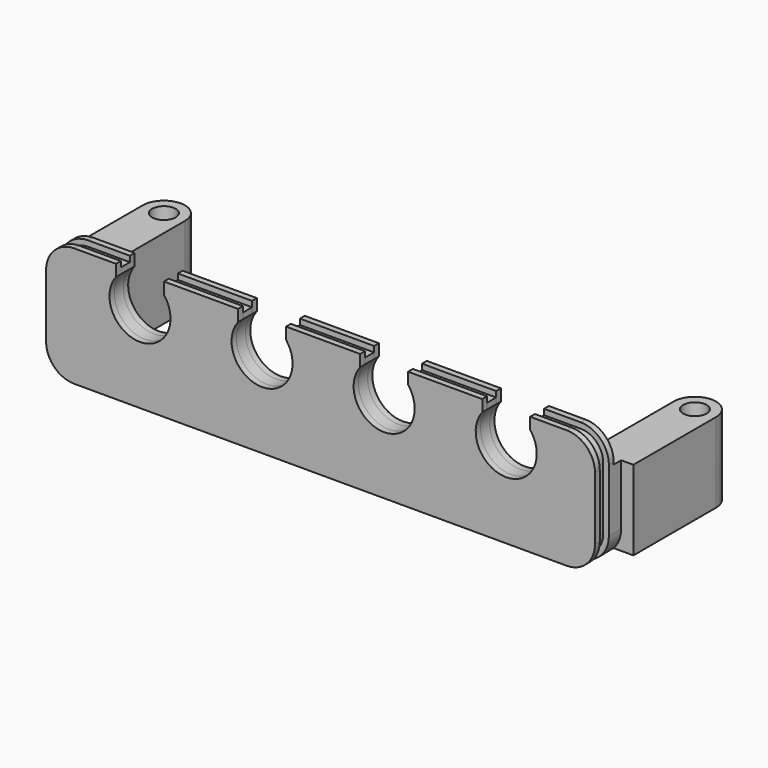
from build123d import *
from build123d import SkipClean  # not in build123d's __all__

# Parameters (mm, degrees)
F1_DEPTH = 0.64
F3_DEPTH = 1.21
F5_DEPTH = 0.64
F7_R     = 1.25
F8_DEPTH = 8.5
F9_DEPTH = 1


# Not quite as in the source:
# - after a boolean that leaves OpenCascade's solid faulty, fix() repairs it


with BuildPart() as f1:
    # F0 (on Front) → F1 (new body)
    with BuildSketch(Plane.XZ):
        with BuildLine():
            ThreePointArc((-29.225, -3.35), (-28.3463203436, -5.4713203436), (-26.225, -6.35))
            Line((-26.225, -6.35), (26.225, -6.35))
            ThreePointArc((26.225, -6.35), (28.3463203436, -5.4713203436), (29.225, -3.35))
            Line((29.225, -3.35), (29.225, 3.35))
            ThreePointArc((29.225, 3.35), (28.3463203436, 5.4713203436), (26.225, 6.35))
            Line((26.225, 6.35), (22.325, 6.35))
            Line((22.325, 6.35), (22.325, 5.114944168))
            ThreePointArc((22.325, 5.114944168), (19.775, -0.15), (17.225, 5.114944168))
            Line((17.225, 5.114944168), (17.225, 6.35))
            Line((17.225, 6.35), (9.325, 6.35))
            Line((9.325, 6.35), (9.325, 5.114944168))
            ThreePointArc((9.325, 5.114944168), (6.775, -0.15), (4.225, 5.114944168))
            Line((4.225, 5.114944168), (4.225, 6.35))
            Line((4.225, 6.35), (-3.675, 6.35))
            Line((-3.675, 6.35), (-3.675, 5.114944168))
            ThreePointArc((-3.675, 5.114944168), (-6.225, -0.15), (-8.775, 5.114944168))
            Line((-8.775, 5.114944168), (-8.775, 6.35))
            Line((-8.775, 6.35), (-16.675, 6.35))
            Line((-16.675, 6.35), (-16.675, 5.114944168))
            ThreePointArc((-16.675, 5.114944168), (-19.225, -0.15), (-21.775, 5.114944168))
            Line((-21.775, 5.114944168), (-21.775, 6.35))
            Line((-21.775, 6.35), (-26.225, 6.35))
            ThreePointArc((-26.225, 6.35), (-28.3463203436, 5.4713203436), (-29.225, 3.35))
            Line((-29.225, 3.35), (-29.225, -3.35))
        make_face()
    extrude(amount=-F1_DEPTH)

    # F2 (on face) → F3 (join)
    with BuildSketch(Plane(origin=(0, 0.64, 0), x_dir=(-1, 0, 0), z_dir=(0, 1, 0))):
        with BuildLine():
            Line((-22.325, 5.114944168), (-22.325, 5.75))
            Line((-22.325, 5.75), (-26.225, 5.75))
            ThreePointArc((-26.225, 5.75), (-27.9220562748, 5.0470562748), (-28.625, 3.35))
            Line((-28.625, 3.35), (-28.625, -3.35))
            ThreePointArc((-28.625, -3.35), (-27.9220562748, -5.0470562748), (-26.225, -5.75))
            Line((-26.225, -5.75), (26.225, -5.75))
            ThreePointArc((26.225, -5.75), (27.9220562748, -5.0470562748), (28.625, -3.35))
            Line((28.625, -3.35), (28.625, 3.35))
            ThreePointArc((28.625, 3.35), (27.9220562748, 5.0470562748), (26.225, 5.75))
            Line((26.225, 5.75), (21.775, 5.75))
            Line((21.775, 5.75), (21.775, 5.114944168))
            ThreePointArc((21.775, 5.114944168), (19.225, -0.15), (16.675, 5.114944168))
            Line((16.675, 5.114944168), (16.675, 5.75))
            Line((16.675, 5.75), (8.775, 5.75))
            Line((8.775, 5.75), (8.775, 5.114944168))
            ThreePointArc((8.775, 5.114944168), (6.225, -0.15), (3.675, 5.114944168))
            Line((3.675, 5.114944168), (3.675, 5.75))
            Line((3.675, 5.75), (-4.225, 5.75))
            Line((-4.225, 5.75), (-4.225, 5.114944168))
            ThreePointArc((-4.225, 5.114944168), (-6.775, -0.15), (-9.325, 5.114944168))
            Line((-9.325, 5.114944168), (-9.325, 5.75))
            Line((-9.325, 5.75), (-17.225, 5.75))
            Line((-17.225, 5.75), (-17.225, 5.114944168))
            ThreePointArc((-17.225, 5.114944168), (-19.775, -0.15), (-22.325, 5.114944168))
        make_face()
    with SkipClean():  # cleaning this boolean's faces spoils the solid; the shape is the same uncleaned
        extrude(amount=F3_DEPTH)

    # F4 (on face) → F5 (join)
    with BuildSketch(Plane(origin=(0, 1.85, 0), x_dir=(-1, 0, 0), z_dir=(0, 1, 0))):
        with BuildLine():
            ThreePointArc((-29.225, -3.35), (-28.3463203436, -5.4713203436), (-26.225, -6.35))
            Line((-26.225, -6.35), (26.225, -6.35))
            ThreePointArc((26.225, -6.35), (28.3463203436, -5.4713203436), (29.225, -3.35))
            Line((29.225, -3.35), (29.225, 3.35))
            ThreePointArc((29.225, 3.35), (28.3463203436, 5.4713203436), (26.225, 6.35))
            Line((26.225, 6.35), (21.775, 6.35))
            Line((21.775, 6.35), (21.775, 5.114944168))
            ThreePointArc((21.775, 5.114944168), (19.225, -0.15), (16.675, 5.114944168))
            Line((16.675, 5.114944168), (16.675, 6.35))
            Line((16.675, 6.35), (8.775, 6.35))
            Line((8.775, 6.35), (8.775, 5.114944168))
            ThreePointArc((8.775, 5.114944168), (6.225, -0.15), (3.675, 5.114944168))
            Line((3.675, 5.114944168), (3.675, 6.35))
            Line((3.675, 6.35), (-4.225, 6.35))
            Line((-4.225, 6.35), (-4.225, 5.114944168))
            ThreePointArc((-4.225, 5.114944168), (-6.775, -0.15), (-9.325, 5.114944168))
            Line((-9.325, 5.114944168), (-9.325, 6.35))
            Line((-9.325, 6.35), (-17.225, 6.35))
            Line((-17.225, 6.35), (-17.225, 5.114944168))
            ThreePointArc((-17.225, 5.114944168), (-19.775, -0.15), (-22.325, 5.114944168))
            Line((-22.325, 5.114944168), (-22.325, 6.35))
            Line((-22.325, 6.35), (-26.225, 6.35))
            ThreePointArc((-26.225, 6.35), (-28.3463203436, 5.4713203436), (-29.225, 3.35))
            Line((-29.225, 3.35), (-29.225, -3.35))
        make_face()
    extrude(amount=F5_DEPTH)

    add(f1.part.fix(), mode=Mode.REPLACE)

    # F7 (on offset) → F8 (join)
    with BuildSketch(Plane(origin=(0, 0, -5.4), x_dir=(1, 0, 0), z_dir=(0, 0, -1))):
        with BuildLine():
            Line((29.225, -3.49), (29.225, -2.49))
            Line((29.225, -2.49), (26.025, -2.49))
            Line((26.025, -2.49), (26.025, -3.49))
            Line((26.025, -3.49), (26.025, -14.49))
            ThreePointArc((26.025, -14.49), (28.275, -16.74), (30.525, -14.49))
            Line((30.525, -14.49), (30.525, -3.49))
            Line((30.525, -3.49), (29.225, -3.49))
        make_face()
        with Locations((28.275, -14.49)):
            Circle(F7_R, mode=Mode.SUBTRACT)
        with BuildLine():
            Line((-26.025, -14.49), (-26.025, -3.49))
            Line((-26.025, -3.49), (-26.025, -2.49))
            Line((-26.025, -2.49), (-29.225, -2.49))
            Line((-29.225, -2.49), (-29.225, -3.49))
            Line((-29.225, -3.49), (-30.525, -3.49))
            Line((-30.525, -3.49), (-30.525, -14.49))
            ThreePointArc((-30.525, -14.49), (-28.275, -16.74), (-26.025, -14.49))
        make_face()
        with Locations((-28.275, -14.49)):
            Circle(F7_R, mode=Mode.SUBTRACT)
    extrude(amount=-F8_DEPTH)

    # F9 (cut): faces of the model
    f9_faces = [f1.faces().sort_by_distance(p)[0] for p in [
        (28.9889729085, 2.49, -4.9023634763),
        (-28.9889729085, 2.49, -4.9023634763),
    ]]
    extrude(f9_faces, amount=-F9_DEPTH, mode=Mode.SUBTRACT)


solid = f1.part
